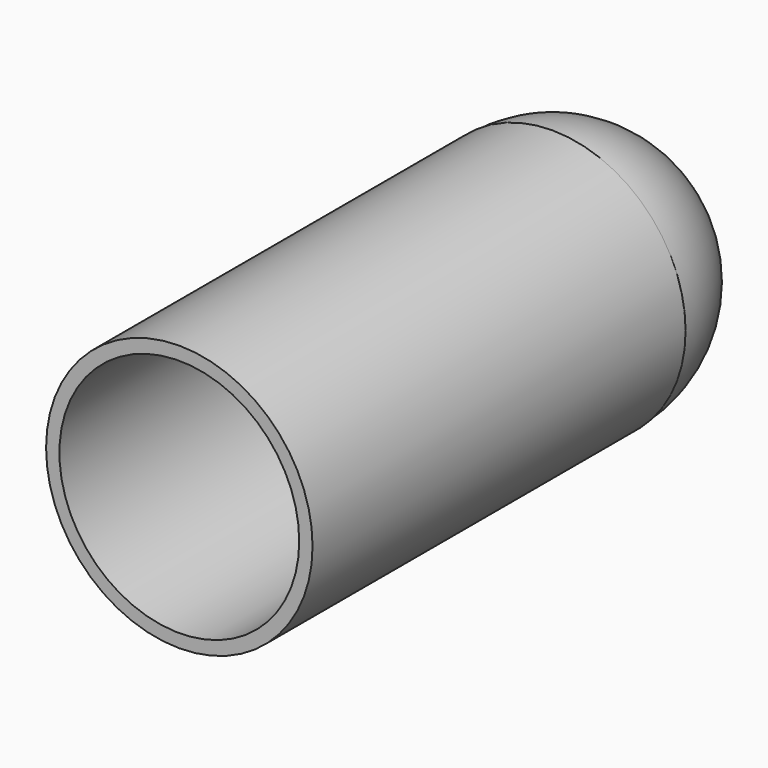
from build123d import *

# Parameters (mm, degrees)
F0_R     = 50
F1_DEPTH = 175
F5_D     = 90
F5_DEPTH = 175.001


with BuildPart() as f1:
    # F0 (on Front) → F1 (new body)
    with BuildSketch(Plane.XZ):
        Circle(F0_R)
    extrude(amount=F1_DEPTH)

    # F2 (on Front) → F3 (revolve)
    with BuildSketch(Plane.XZ):
        with BuildLine():
            Line((0, -49.6900500015), (0, 49.6900500015))
            ThreePointArc((0, 49.6900500015), (-49.6900500015, 0), (0, -49.6900500015))
        make_face()
    revolve(axis=Axis((0, 0, 0), (0, 0, -1)))

    # F5 (through all, one way)
    with BuildSketch(Plane(origin=(0, 0, 0), x_dir=(1, 0, 0), z_dir=(0, 1, 0))):
        with Locations((0, 0)):
            Circle(F5_D / 2)
    extrude(amount=-F5_DEPTH, mode=Mode.SUBTRACT)


solid = f1.part
